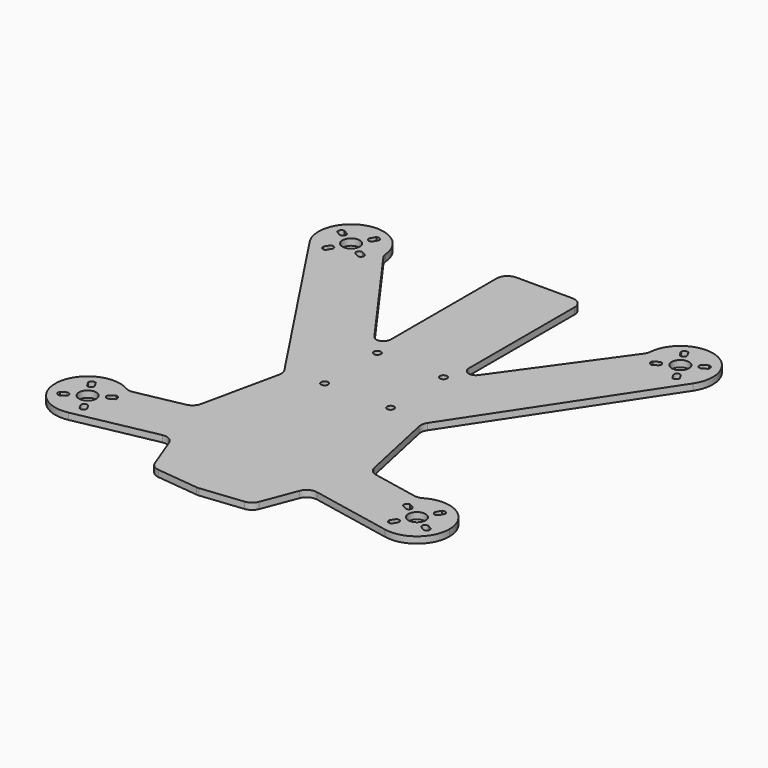
from build123d import *

# Parameters (mm, degrees)
F0_R        = 4
F0_R_2      = 1.6
F1_DEPTH    = 3
F2_R        = 5
F3_T1_DEPTH = 3


# Not quite as in the source:
# - a fillet or chamfer that OpenCascade refuses, or shapes differently, is made with other operations: its cross-section is extruded or revolved along the edge and cut away or added


with BuildPart() as f1:
    # F0 (on Top) → F1 (new body)
    with BuildSketch(Plane.XY):
        with BuildLine():
            ThreePointArc((-88.527031831, 67.7421286231), (-71.6951708551, 61.6491644503), (-61.0139789776, 76.0139789776))
            ThreePointArc((-61.0139789776, 76.0139789776), (-80.3327871, 90.3787935048), (-88.527031831, 67.7421286231))
        make_face()
        with BuildLine():
            ThreePointArc((-81.2139789776, 69.7785960703), (-79.3211586545, 70.2857757473), (-78.8139789776, 68.3929554243))
            Line((-78.8139789776, 68.3929554243), (-79.9639789776, 66.4010969955))
            ThreePointArc((-79.9639789776, 66.4010969955), (-81.5639789776, 66.4010969955), (-82.3639789776, 67.7867376416))
            Line((-82.3639789776, 67.7867376416), (-81.2139789776, 69.7785960703))
        make_face(mode=Mode.SUBTRACT)
        with BuildLine():
            ThreePointArc((-69.7785960703, 70.8139789776), (-70.2857757473, 72.7067993006), (-68.3929554243, 73.2139789776))
            Line((-68.3929554243, 73.2139789776), (-66.4010969955, 72.0639789776))
            ThreePointArc((-66.4010969955, 72.0639789776), (-66.4010969955, 70.4639789776), (-67.7867376416, 69.6639789776))
            Line((-67.7867376416, 69.6639789776), (-69.7785960703, 70.8139789776))
        make_face(mode=Mode.SUBTRACT)
        with Locations((-76.0139789776, 76.0139789776)):
            Circle(F0_R, mode=Mode.SUBTRACT)
        with BuildLine():
            ThreePointArc((-82.2493618848, 81.2139789776), (-81.7421822078, 79.3211586545), (-83.6350025309, 78.8139789776))
            Line((-83.6350025309, 78.8139789776), (-85.6268609596, 79.9639789776))
            ThreePointArc((-85.6268609596, 79.9639789776), (-85.6268609596, 81.5639789776), (-84.2412203135, 82.3639789776))
            Line((-84.2412203135, 82.3639789776), (-82.2493618848, 81.2139789776))
        make_face(mode=Mode.SUBTRACT)
        with BuildLine():
            ThreePointArc((-70.8139789776, 82.2493618848), (-72.7067993006, 81.7421822078), (-73.2139789776, 83.6350025309))
            Line((-73.2139789776, 83.6350025309), (-72.0639789776, 85.6268609596))
            ThreePointArc((-72.0639789776, 85.6268609596), (-70.4639789776, 85.6268609596), (-69.6639789776, 84.2412203135))
            Line((-69.6639789776, 84.2412203135), (-70.8139789776, 82.2493618848))
        make_face(mode=Mode.SUBTRACT)
        with BuildLine():
            Line((-23, 23), (-61.0139789776, 76.0139789776))
            ThreePointArc((-61.0139789776, 76.0139789776), (-71.6951708551, 61.6491644503), (-88.527031831, 67.7421286231))
            Line((-88.527031831, 67.7421286231), (-31.8465346459, -18))
            Line((-31.8465346459, -18), (-40.6432183342, -58.7689615944))
            Line((-40.6432183342, -58.7689615944), (-67.0035176261, -64.0218321208))
            ThreePointArc((-67.0035176261, -64.0218321208), (-62.5946473945, -69.3116256696), (-61.0139789776, -76.0139789776))
            ThreePointArc((-61.0139789776, -76.0139789776), (-64.4171763077, -85.5278723886), (-73.0825346892, -90.7247449122))
            Line((-73.0825346892, -90.7247449122), (-31.6043349446, -82.4592995729))
            Line((-31.6043349446, -82.4592995729), (-23, -105.0107137391))
            Line((-23, -105.0107137391), (0, -107.5))
            Line((0, -107.5), (23, -105.0107137391))
            Line((23, -105.0107137391), (31.6043349446, -82.4592995729))
            Line((31.6043349446, -82.4592995729), (73.0825346892, -90.7247449122))
            ThreePointArc((73.0825346892, -90.7247449122), (61.3881912906, -79.3435937504), (67.0035176261, -64.0218321208))
            Line((67.0035176261, -64.0218321208), (40.6432183342, -58.7689615944))
            Line((40.6432183342, -58.7689615944), (31.8465346459, -18))
            Line((31.8465346459, -18), (88.527031831, 67.7421286231))
            ThreePointArc((88.527031831, 67.7421286231), (71.6951708551, 61.6491644503), (61.0139789776, 76.0139789776))
            Line((61.0139789776, 76.0139789776), (23, 23))
            Line((23, 23), (18, 23))
            Line((18, 23), (18, 92.5))
            Line((18, 92.5), (0, 92.5))
            Line((0, 92.5), (-18, 92.5))
            Line((-18, 92.5), (-18, 23))
            Line((-18, 23), (-23, 23))
        make_face()
        with Locations((-15.25, -15.25)):
            Circle(F0_R_2, mode=Mode.SUBTRACT)
        with Locations((15.25, -15.25)):
            Circle(F0_R_2, mode=Mode.SUBTRACT)
        with Locations((-15.25, 15.25)):
            Circle(F0_R_2, mode=Mode.SUBTRACT)
        with Locations((15.25, 15.25)):
            Circle(F0_R_2, mode=Mode.SUBTRACT)
        with BuildLine():
            ThreePointArc((-61.0139789776, -76.0139789776), (-62.5946473945, -69.3116256696), (-67.0035176261, -64.0218321208))
            ThreePointArc((-67.0035176261, -64.0218321208), (-90.6397666645, -72.6843642047), (-73.0825346892, -90.7247449122))
            ThreePointArc((-73.0825346892, -90.7247449122), (-64.4171763077, -85.5278723886), (-61.0139789776, -76.0139789776))
        make_face()
        with BuildLine():
            Line((-70.8139789776, -82.2493618848), (-69.6639789776, -84.2412203135))
            ThreePointArc((-69.6639789776, -84.2412203135), (-70.4639789776, -85.6268609596), (-72.0639789776, -85.6268609596))
            Line((-72.0639789776, -85.6268609596), (-73.2139789776, -83.6350025309))
            ThreePointArc((-73.2139789776, -83.6350025309), (-72.7067993006, -81.7421822078), (-70.8139789776, -82.2493618848))
        make_face(mode=Mode.SUBTRACT)
        with BuildLine():
            Line((-85.6268609596, -79.9639789776), (-83.6350025309, -78.8139789776))
            ThreePointArc((-83.6350025309, -78.8139789776), (-81.7421822078, -79.3211586545), (-82.2493618848, -81.2139789776))
            Line((-82.2493618848, -81.2139789776), (-84.2412203135, -82.3639789776))
            ThreePointArc((-84.2412203135, -82.3639789776), (-85.6268609596, -81.5639789776), (-85.6268609596, -79.9639789776))
        make_face(mode=Mode.SUBTRACT)
        with Locations((-76.0139789776, -76.0139789776)):
            Circle(F0_R, mode=Mode.SUBTRACT)
        with BuildLine():
            Line((-66.4010969955, -72.0639789776), (-68.3929554243, -73.2139789776))
            ThreePointArc((-68.3929554243, -73.2139789776), (-70.2857757473, -72.7067993006), (-69.7785960703, -70.8139789776))
            Line((-69.7785960703, -70.8139789776), (-67.7867376416, -69.6639789776))
            ThreePointArc((-67.7867376416, -69.6639789776), (-66.4010969955, -70.4639789776), (-66.4010969955, -72.0639789776))
        make_face(mode=Mode.SUBTRACT)
        with BuildLine():
            Line((-79.9639789776, -66.4010969955), (-78.8139789776, -68.3929554243))
            ThreePointArc((-78.8139789776, -68.3929554243), (-79.3211586545, -70.2857757473), (-81.2139789776, -69.7785960703))
            Line((-81.2139789776, -69.7785960703), (-82.3639789776, -67.7867376416))
            ThreePointArc((-82.3639789776, -67.7867376416), (-81.5639789776, -66.4010969955), (-79.9639789776, -66.4010969955))
        make_face(mode=Mode.SUBTRACT)
        with BuildLine():
            ThreePointArc((91.0139789776, 76.0139789776), (76.0139789776, 91.0139789776), (61.0139789776, 76.0139789776))
            ThreePointArc((61.0139789776, 76.0139789776), (71.6951708551, 61.6491644503), (88.527031831, 67.7421286231))
            ThreePointArc((88.527031831, 67.7421286231), (90.3787935048, 71.6951708551), (91.0139789776, 76.0139789776))
        make_face()
        with BuildLine():
            Line((66.4010969955, 72.0639789776), (68.3929554243, 73.2139789776))
            ThreePointArc((68.3929554243, 73.2139789776), (70.2857757473, 72.7067993006), (69.7785960703, 70.8139789776))
            Line((69.7785960703, 70.8139789776), (67.7867376416, 69.6639789776))
            ThreePointArc((67.7867376416, 69.6639789776), (66.4010969955, 70.4639789776), (66.4010969955, 72.0639789776))
        make_face(mode=Mode.SUBTRACT)
        with Locations((76.0139789776, 76.0139789776)):
            Circle(F0_R, mode=Mode.SUBTRACT)
        with BuildLine():
            Line((79.9639789776, 66.4010969955), (78.8139789776, 68.3929554243))
            ThreePointArc((78.8139789776, 68.3929554243), (79.3211586545, 70.2857757473), (81.2139789776, 69.7785960703))
            Line((81.2139789776, 69.7785960703), (82.3639789776, 67.7867376416))
            ThreePointArc((82.3639789776, 67.7867376416), (81.5639789776, 66.4010969955), (79.9639789776, 66.4010969955))
        make_face(mode=Mode.SUBTRACT)
        with BuildLine():
            ThreePointArc((73.2139789776, 83.6350025309), (72.7067993006, 81.7421822078), (70.8139789776, 82.2493618848))
            Line((70.8139789776, 82.2493618848), (69.6639789776, 84.2412203135))
            ThreePointArc((69.6639789776, 84.2412203135), (70.4639789776, 85.6268609596), (72.0639789776, 85.6268609596))
            Line((72.0639789776, 85.6268609596), (73.2139789776, 83.6350025309))
        make_face(mode=Mode.SUBTRACT)
        with BuildLine():
            Line((85.6268609596, 79.9639789776), (83.6350025309, 78.8139789776))
            ThreePointArc((83.6350025309, 78.8139789776), (81.7421822078, 79.3211586545), (82.2493618848, 81.2139789776))
            Line((82.2493618848, 81.2139789776), (84.2412203135, 82.3639789776))
            ThreePointArc((84.2412203135, 82.3639789776), (85.6268609596, 81.5639789776), (85.6268609596, 79.9639789776))
        make_face(mode=Mode.SUBTRACT)
        with BuildLine():
            ThreePointArc((67.0035176261, -64.0218321208), (61.3881912906, -79.3435937504), (73.0825346892, -90.7247449122))
            ThreePointArc((73.0825346892, -90.7247449122), (85.5278723886, -87.6107816474), (91.0139789776, -76.0139789776))
            ThreePointArc((91.0139789776, -76.0139789776), (82.7163322855, -62.5946473945), (67.0035176261, -64.0218321208))
        make_face()
        with BuildLine():
            ThreePointArc((70.8139789776, -82.2493618848), (72.7067993006, -81.7421822078), (73.2139789776, -83.6350025309))
            Line((73.2139789776, -83.6350025309), (72.0639789776, -85.6268609596))
            ThreePointArc((72.0639789776, -85.6268609596), (70.4639789776, -85.6268609596), (69.6639789776, -84.2412203135))
            Line((69.6639789776, -84.2412203135), (70.8139789776, -82.2493618848))
        make_face(mode=Mode.SUBTRACT)
        with BuildLine():
            ThreePointArc((69.7785960703, -70.8139789776), (70.2857757473, -72.7067993006), (68.3929554243, -73.2139789776))
            Line((68.3929554243, -73.2139789776), (66.4010969955, -72.0639789776))
            ThreePointArc((66.4010969955, -72.0639789776), (66.4010969955, -70.4639789776), (67.7867376416, -69.6639789776))
            Line((67.7867376416, -69.6639789776), (69.7785960703, -70.8139789776))
        make_face(mode=Mode.SUBTRACT)
        with Locations((76.0139789776, -76.0139789776)):
            Circle(F0_R, mode=Mode.SUBTRACT)
        with BuildLine():
            ThreePointArc((82.2493618848, -81.2139789776), (81.7421822078, -79.3211586545), (83.6350025309, -78.8139789776))
            Line((83.6350025309, -78.8139789776), (85.6268609596, -79.9639789776))
            ThreePointArc((85.6268609596, -79.9639789776), (85.6268609596, -81.5639789776), (84.2412203135, -82.3639789776))
            Line((84.2412203135, -82.3639789776), (82.2493618848, -81.2139789776))
        make_face(mode=Mode.SUBTRACT)
        with BuildLine():
            ThreePointArc((81.2139789776, -69.7785960703), (79.3211586545, -70.2857757473), (78.8139789776, -68.3929554243))
            Line((78.8139789776, -68.3929554243), (79.9639789776, -66.4010969955))
            ThreePointArc((79.9639789776, -66.4010969955), (81.5639789776, -66.4010969955), (82.3639789776, -67.7867376416))
            Line((82.3639789776, -67.7867376416), (81.2139789776, -69.7785960703))
        make_face(mode=Mode.SUBTRACT)
    extrude(amount=F1_DEPTH)

    # F2
    f2_edges = [f1.edges().sort_by_distance(p)[0] for p in [
        (-31.846535, -18, 1.5),
        (31.846535, -18, 1.5),
        (40.643218, -58.768962, 1.5),
        (-40.643218, -58.768962, 1.5),
        (-31.604335, -82.4593, 1.5),
        (31.604335, -82.4593, 1.5),
        (23, -105.010714, 1.5),
        (-23, -105.010714, 1.5),
        (0, -107.5, 1.5),
        (67.003518, -64.021832, 1.5),
        (-67.003518, -64.021832, 1.5),
        (61.013979, 76.013979, 1.5),
        (-61.013979, 76.013979, 1.5),
        (18, 92.5, 1.5),
        (-18, 92.5, 1.5),
    ]]
    fillet(f2_edges, radius=F2_R)

    # F3: fillet of radius 3.5 on 4 edges, made by hand

    # F3_s2 → F3_t1 (join)
    with BuildSketch(Plane.XY):
        with BuildLine():
            ThreePointArc((-24.0472259483, 24.4604525993), (-22.8015745775, 23.3864476958), (-21.2028901031, 23))
            Line((-21.2028901031, 23), (-23, 23))
            Line((-23, 23), (-24.0472259483, 24.4604525993))
        make_face()
        with BuildLine():
            ThreePointArc((-21.5, 23), (-19.0251262658, 24.0251262658), (-18, 26.5))
            Line((-18, 26.5), (-18, 23))
            Line((-18, 23), (-21.5, 23))
        make_face()
        with BuildLine():
            ThreePointArc((18, 26.5), (19.0251262658, 24.0251262658), (21.5, 23))
            Line((21.5, 23), (18, 23))
            Line((18, 23), (18, 26.5))
        make_face()
        with BuildLine():
            ThreePointArc((21.2028901031, 23), (22.8015745775, 23.3864476958), (24.0472259483, 24.4604525993))
            Line((24.0472259483, 24.4604525993), (23, 23))
            Line((23, 23), (21.2028901031, 23))
        make_face()
    extrude(amount=F3_T1_DEPTH)


solid = f1.part
